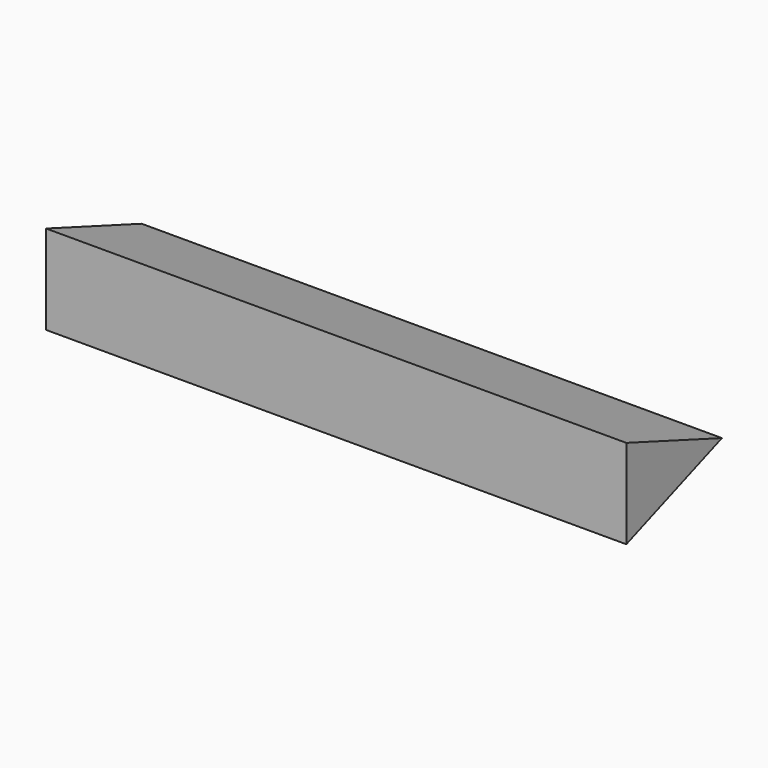
from build123d import *

# Parameters (mm, degrees)
F3_DEPTH = 16.51


# Not quite as in the source:
# - the program builds the solid bodies; features that only make, move or delete a surface that nothing else refers to are left out


with BuildPart() as f3:
    # F2 (on Right) → F3 (new body, symmetric)
    with BuildSketch(Plane.YZ):
        Polygon((6.7997026871, 0), (0, 2.5235276793), (0, -2.5564723207), align=None)
    extrude(amount=F3_DEPTH, both=True)


solid = f3.part
